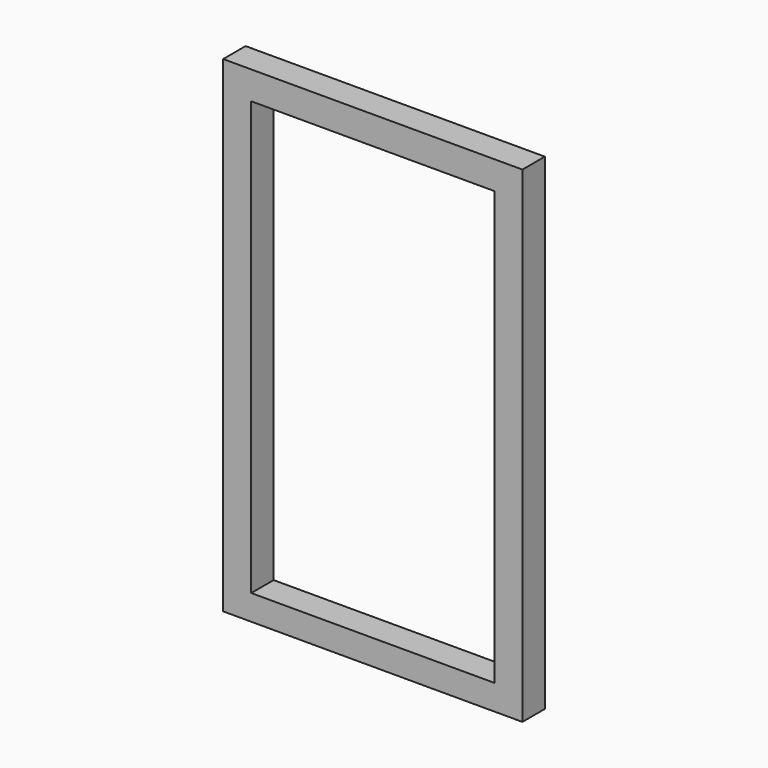
from build123d import *

# Parameters (mm, degrees)
F0_W     = 38.1
F0_H     = 38.1
F1_DEPTH = 660.4
F2_W     = 38.1
F2_H     = 38.1
F3_DEPTH = 330.2
F4_W     = 38.1
F4_H     = 34.3169383705
F5_DEPTH = 330.2
F6_W     = 38.1
F6_H     = 38.1
F7_DEPTH = 660.4


with BuildPart() as f1:
    # F0 (on Top) → F1 (new body)
    with BuildSketch(Plane.XY):
        Rectangle(F0_W, F0_H)
    extrude(amount=F1_DEPTH)

    # F2 (on face) → F3 (join)
    with BuildSketch(Plane.YZ.offset(19.05)):
        with Locations((0, 641.35)):
            Rectangle(F2_W, F2_H)
    extrude(amount=F3_DEPTH)

    # F4 (on face) → F5 (join)
    with BuildSketch(Plane.YZ.offset(19.05)):
        with Locations((0, 17.1584691852)):
            Rectangle(F4_W, F4_H)
    extrude(amount=F5_DEPTH)

    # F6 (on face) → F7 (join)
    with BuildSketch(Plane(origin=(0, 0, 0), x_dir=(1, 0, 0), z_dir=(0, 0, -1))):
        with Locations((368.3, 0)):
            Rectangle(F6_W, F6_H)
    extrude(amount=-F7_DEPTH)


solid = f1.part
